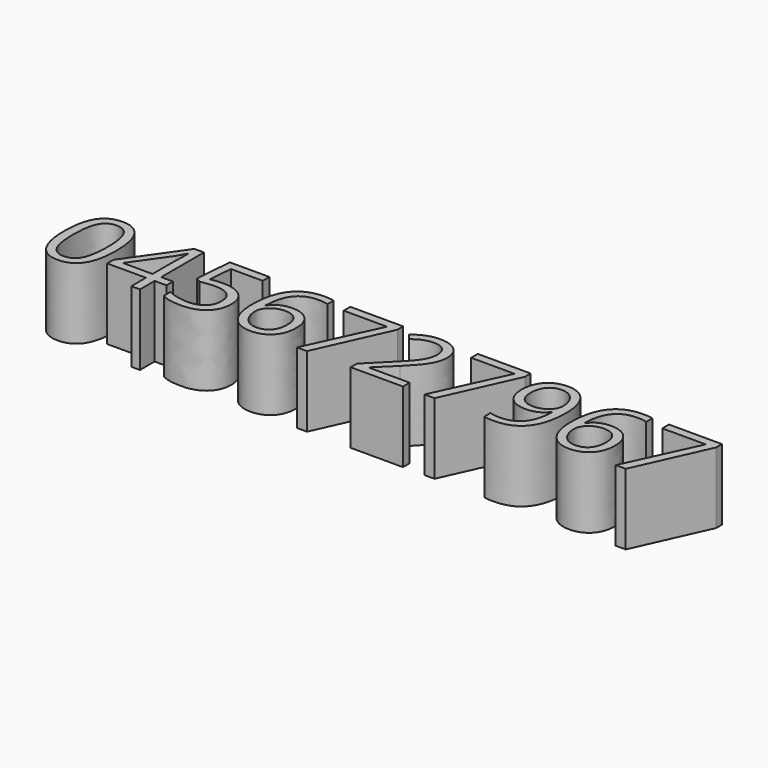
from build123d import *

# Parameters (mm, degrees)
F0_TEXT_SIZE = 15.7033805889
F1_DEPTH     = 10


# Not quite as in the source:
# - a feature of the source that left no trace in its solid (it failed there, or was rolled back) is left out
# - Text() gives the source's letters only with a copy of the font that has no kerning and outlines rounded to 1/6400 em; it was checked with that copy


with BuildPart() as f1:
    # F0 (on Top) → F1 (new body)
    with BuildSketch(Plane.XY):
        with Locations((-45, -5.653217012)):
            Text('0456727967', F0_TEXT_SIZE, font='Open Sans', text_align=(TextAlign.LEFT, TextAlign.BOTTOM))
    extrude(amount=F1_DEPTH)


solid = f1.part
